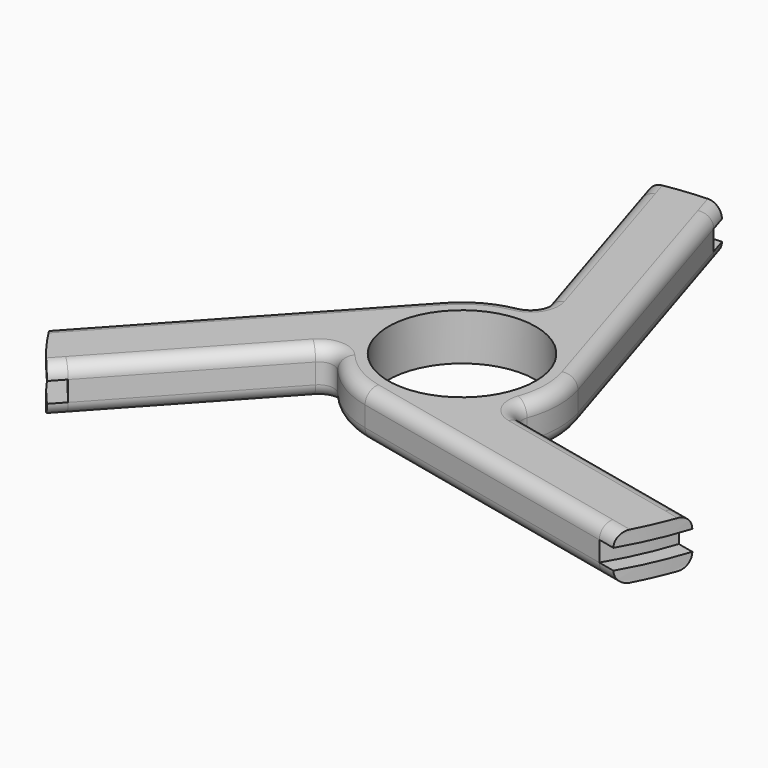
from build123d import *

# Parameters (mm, degrees)
F0_R     = 11
F1_DEPTH = 3.5
F2_R     = 2
F3_R     = 2
F4_DEPTH = 1.5


with BuildPart() as f1:
    # F0 (on Top) → F1 (new body, symmetric)
    with BuildSketch(Plane.XY):
        with BuildLine():
            ThreePointArc((-0.8285496132, 17.1446015607), (-1.0500524725, 15.314704152), (-2.5690728422, 14.2705944071))
            ThreePointArc((-2.5690728422, 14.2705944071), (-6.985549163, 12.7063804009), (-10.6726700751, 9.8155037297))
            Line((-10.6726700751, 9.8155037297), (-40.2240356418, -22.3165175753))
            ThreePointArc((-40.2240356418, -22.3165175753), (-37.447016124, -26.7155569548), (-34.1910537852, -30.7729075821))
            Line((-34.1910537852, -30.7729075821), (-14.4333856827, -9.2898457936))
            ThreePointArc((-14.4333856827, -9.2898457936), (-12.7378966108, -8.5667241925), (-11.0741608625, -9.3601795491))
            ThreePointArc((-11.0741608625, -9.3601795491), (-7.5112736358, -12.4028532349), (-3.1641405433, -14.1505552761))
            Line((-3.1641405433, -14.1505552761), (39.4386889651, -23.6767779209))
            ThreePointArc((39.4386889651, -23.6767779209), (41.8598590611, -19.0722887819), (43.745646607, -14.2238673691))
            Line((43.745646607, -14.2238673691), (15.2619352959, -7.8547557671))
            ThreePointArc((15.2619352959, -7.8547557671), (13.7879490833, -6.7479799595), (13.6432337047, -4.910414858))
            ThreePointArc((13.6432337047, -4.910414858), (14.4968227988, -0.3035271659), (13.8368106184, 4.3350515464))
            Line((13.8368106184, 4.3350515464), (0.7853466767, 45.9932954962))
            ThreePointArc((0.7853466767, 45.9932954962), (-4.4128429371, 45.7878457368), (-9.5545928219, 44.9967749512))
            Line((-9.5545928219, 44.9967749512), (-0.8285496132, 17.1446015607))
        make_face()
        Circle(F0_R, mode=Mode.SUBTRACT)
        with BuildLine():
            Line((-10.3051834804, 47.3925436481), (-9.5545928219, 44.9967749512))
            ThreePointArc((-9.5545928219, 44.9967749512), (-4.4128429371, 45.7878457368), (0.7853466767, 45.9932954962))
            Line((0.7853466767, 45.9932954962), (0, 48.5))
            ThreePointArc((0, 48.5), (-5.1822597903, 48.2223411239), (-10.3051834804, 47.3925436481))
        make_face()
        with BuildLine():
            ThreePointArc((43.745646607, -14.2238673691), (41.8598590611, -19.0722887819), (39.4386889651, -23.6767779209))
            Line((39.4386889651, -23.6767779209), (42.0022320835, -24.25))
            ThreePointArc((42.0022320835, -24.25), (44.3529023384, -19.6232019345), (46.1957384894, -14.7717211394))
            Line((46.1957384894, -14.7717211394), (43.745646607, -14.2238673691))
        make_face()
        with BuildLine():
            ThreePointArc((-34.1910537852, -30.7729075821), (-37.447016124, -26.7155569548), (-40.2240356418, -22.3165175753))
            Line((-40.2240356418, -22.3165175753), (-42.0022320835, -24.25))
            ThreePointArc((-42.0022320835, -24.25), (-39.1706425481, -28.5991391893), (-35.890555009, -32.6208225087))
            Line((-35.890555009, -32.6208225087), (-34.1910537852, -30.7729075821))
        make_face()
    extrude(amount=F1_DEPTH, both=True)

    # F2
    f2_edges = [f1.edges().sort_by_distance(p)[0] for p in [
        (-26.337451, -7.217248, 3.5),
        (-6.985549, 12.70638, 3.5),
        (-1.050052, 15.314704, 3.5),
        (-5.566867, 32.268573, 3.5),
        (6.918405, 26.417526, 3.5),
        (14.496823, -0.303527, 3.5),
        (13.787949, -6.74798, 3.5),
        (30.728837, -11.313238, 3.5),
        (19.419046, -19.200278, 3.5),
        (-7.511274, -12.402853, 3.5),
        (-12.737897, -8.566724, 3.5),
        (-25.16197, -20.955334, 3.5),
    ]]
    fillet(f2_edges, radius=F2_R)

    # F3
    f3_edges = [f1.edges().sort_by_distance(p)[0] for p in [
        (-26.337451, -7.217248, -3.5),
        (-6.985549, 12.70638, -3.5),
        (-1.050052, 15.314704, -3.5),
        (-5.566867, 32.268573, -3.5),
        (6.918405, 26.417526, -3.5),
        (14.496823, -0.303527, -3.5),
        (13.787949, -6.74798, -3.5),
        (30.728837, -11.313238, -3.5),
        (19.419046, -19.200278, -3.5),
        (-7.511274, -12.402853, -3.5),
        (-12.737897, -8.566724, -3.5),
        (-25.16197, -20.955334, -3.5),
    ]]
    fillet(f3_edges, radius=F3_R)


with BuildPart() as f4:
    # F0 (on Top) → F4 (new body, symmetric)
    with BuildSketch(Plane.XY):
        with BuildLine():
            Line((-10.3051834804, 47.3925436481), (-9.5545928219, 44.9967749512))
            ThreePointArc((-9.5545928219, 44.9967749512), (-4.4128429371, 45.7878457368), (0.7853466767, 45.9932954962))
            Line((0.7853466767, 45.9932954962), (0, 48.5))
            ThreePointArc((0, 48.5), (-5.1822597903, 48.2223411239), (-10.3051834804, 47.3925436481))
        make_face()
        with BuildLine():
            Line((-42.0022320835, -24.25), (-40.2240356418, -22.3165175753))
            ThreePointArc((-40.2240356418, -22.3165175753), (-41.8598590611, 19.0722887819), (-9.5545928219, 44.9967749512))
            Line((-9.5545928219, 44.9967749512), (-10.3051834804, 47.3925436481))
            ThreePointArc((-10.3051834804, 47.3925436481), (-44.3529023384, 19.6232019345), (-42.0022320835, -24.25))
        make_face()
        with BuildLine():
            ThreePointArc((-34.1910537852, -30.7729075821), (-37.447016124, -26.7155569548), (-40.2240356418, -22.3165175753))
            Line((-40.2240356418, -22.3165175753), (-42.0022320835, -24.25))
            ThreePointArc((-42.0022320835, -24.25), (-39.1706425481, -28.5991391893), (-35.890555009, -32.6208225087))
            Line((-35.890555009, -32.6208225087), (-34.1910537852, -30.7729075821))
        make_face()
        with BuildLine():
            ThreePointArc((39.4386889651, -23.6767779209), (4.4128429371, -45.7878457368), (-34.1910537852, -30.7729075821))
            Line((-34.1910537852, -30.7729075821), (-35.890555009, -32.6208225087))
            ThreePointArc((-35.890555009, -32.6208225087), (5.1822597903, -48.2223411239), (42.0022320835, -24.25))
            Line((42.0022320835, -24.25), (39.4386889651, -23.6767779209))
        make_face()
        with BuildLine():
            ThreePointArc((43.745646607, -14.2238673691), (41.8598590611, -19.0722887819), (39.4386889651, -23.6767779209))
            Line((39.4386889651, -23.6767779209), (42.0022320835, -24.25))
            ThreePointArc((42.0022320835, -24.25), (44.3529023384, -19.6232019345), (46.1957384894, -14.7717211394))
            Line((46.1957384894, -14.7717211394), (43.745646607, -14.2238673691))
        make_face()
        with BuildLine():
            Line((0, 48.5), (0.7853466767, 45.9932954962))
            ThreePointArc((0.7853466767, 45.9932954962), (32.8033988112, 32.2480546147), (46, 0))
            ThreePointArc((46, 0), (45.4329161728, -7.2007033016), (43.745646607, -14.2238673691))
            Line((43.745646607, -14.2238673691), (46.1957384894, -14.7717211394))
            ThreePointArc((46.1957384894, -14.7717211394), (47.9204722261, -7.4751817123), (48.5, 0))
            ThreePointArc((48.5, 0), (34.2946788875, 34.2946788875), (0, 48.5))
        make_face()
    extrude(amount=F4_DEPTH, both=True)


with BuildPart() as f1_1:
    add(f1.part)

    # F5: cut F4
    add(f4.part, mode=Mode.SUBTRACT)


solid = f1_1.part
